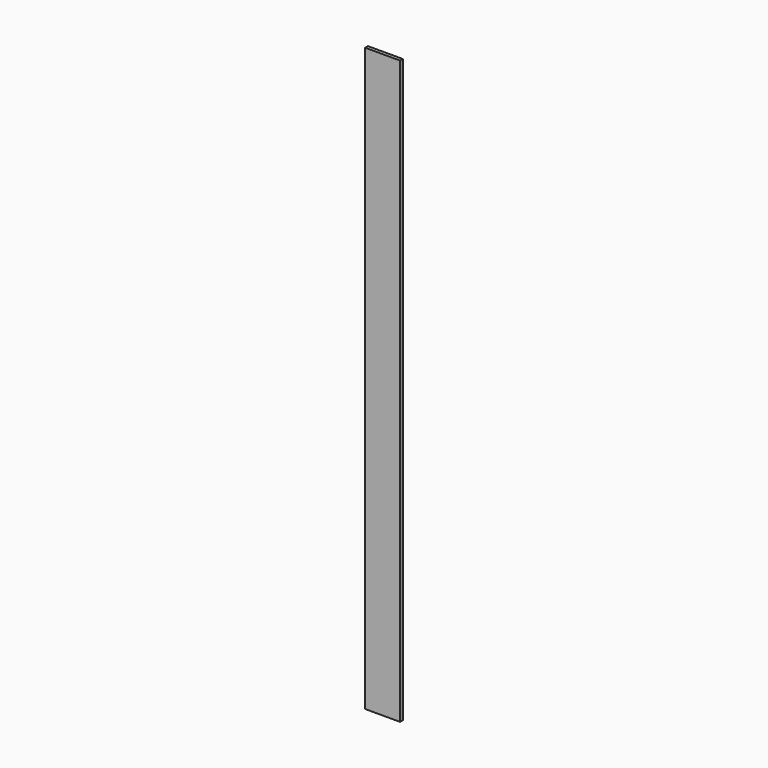
from build123d import *

# Parameters (mm, degrees)
F0_W     = 30
F0_H     = 500
F1_DEPTH = 3
F2_R     = 4.5
F3_DEPTH = 752


# Not quite as in the source:
# - an extrude ends at something that could not be found from the text; its depth is read off the source's solid


with BuildPart() as f1:
    # F0 (on Front) → F1 (new body)
    with BuildSketch(Plane.XZ):
        with Locations((15, 250)):
            Rectangle(F0_W, F0_H)
    extrude(amount=F1_DEPTH)

    # F2 (on face) → F3 (cut, through all)
    with BuildSketch(Plane.XZ):
        with Locations((15, 470)):
            Circle(F2_R)
    extrude(amount=-F3_DEPTH, mode=Mode.SUBTRACT)


solid = f1.part
